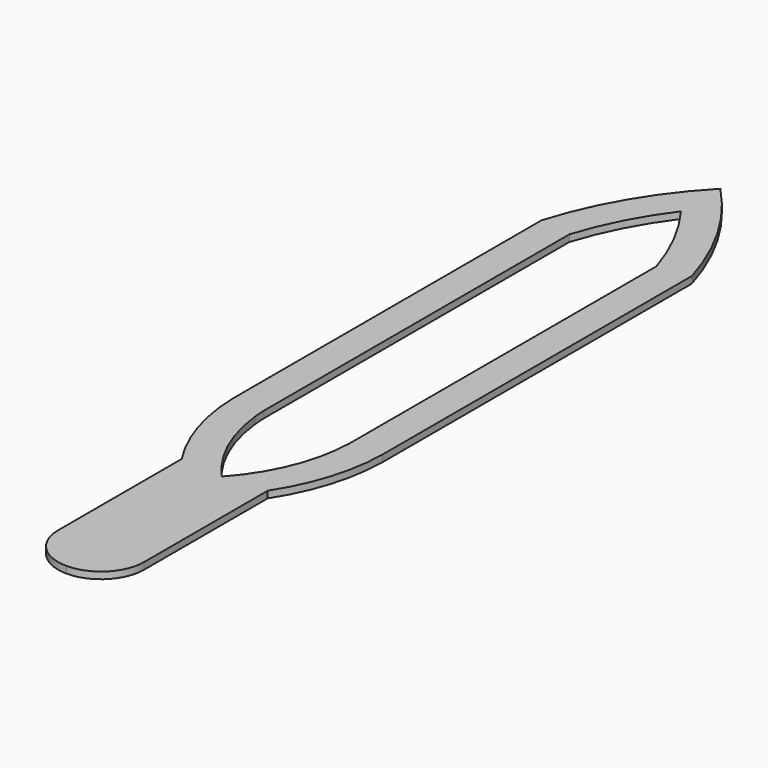
from build123d import *

# Parameters (mm, degrees)
F1_DEPTH = 4
F2_R     = 25.39999


# Not quite as in the source:
# - a fillet or chamfer is up to 0.001 mm smaller than in the source, because OpenCascade refuses the exact size


with BuildPart() as f1:
    # F0 (on Top) → F1 (new body)
    with BuildSketch(Plane.XY):
        with BuildLine():
            Line((25.4, 88.9), (25.4, 27.783106151))
            ThreePointArc((25.4, 27.783106151), (39.0875817391, 57.0211124393), (44.1814440725, 88.9))
            Line((44.1814440725, 88.9), (44.1814440725, 317.5))
            ThreePointArc((44.1814440725, 317.5), (26.6541395651, 358.2459104505), (0, 393.7))
            ThreePointArc((0, 393.7), (-26.9370466698, 358.2864987651), (-44.7185559275, 317.5))
            Line((-44.7185559275, 317.5), (-44.7185559275, 88.9))
            ThreePointArc((-44.7185559275, 88.9), (-39.2808523641, 57.0071475451), (-25.4, 27.783106151))
            Line((-25.4, 27.783106151), (-25.4, 81.8970223493))
            ThreePointArc((-25.4, 81.8970223493), (-25.7287156311, 85.5486031353), (-25.9225594861, 89.209821616))
            Line((-25.9225594861, 89.209821616), (-25.9225594861, 314.6655596019))
            ThreePointArc((-25.9225594861, 314.6655596019), (-15.1225925717, 340.7930484479), (-0.0869368678, 364.7349367673))
            ThreePointArc((-0.0869368678, 364.7349367673), (14.7574318658, 340.7960081036), (25.385447631, 314.7101331987))
            Line((25.385447631, 314.7101331987), (25.385447631, 89.0840377413))
            ThreePointArc((25.385447631, 89.0840377413), (25.3835184902, 88.992017936), (25.3815021522, 88.9))
            Line((25.3815021522, 88.9), (25.4, 88.9))
        make_face()
        with BuildLine():
            Line((-25.4, -88.9), (25.4, -88.9))
            Line((25.4, -88.9), (25.4, 27.783106151))
            ThreePointArc((25.4, 27.783106151), (13.8352633227, 12.8536673819), (0, 0))
            ThreePointArc((0, 0), (-13.8130547318, 12.8739710228), (-25.4, 27.783106151))
            Line((-25.4, 27.783106151), (-25.4, -88.9))
        make_face()
        with BuildLine():
            ThreePointArc((0, 0), (13.8352633227, 12.8536673819), (25.4, 27.783106151))
            Line((25.4, 27.783106151), (25.4, 88.9))
            Line((25.4, 88.9), (25.3815021522, 88.9))
            ThreePointArc((25.3815021522, 88.9), (18.4387554256, 54.950742752), (0.0203713554, 25.5991341412))
            ThreePointArc((0.0203713554, 25.5991341412), (-17.1734173627, 51.7235821598), (-25.4, 81.8970223493))
            Line((-25.4, 81.8970223493), (-25.4, 27.783106151))
            ThreePointArc((-25.4, 27.783106151), (-13.8130547318, 12.8739710228), (0, 0))
        make_face()
    extrude(amount=F1_DEPTH)

    # F2 (radius 25.4 in the source; OpenCascade refuses exactly that, so slightly less here)
    f2_edges = [f1.edges().sort_by_distance(p)[0] for p in [
        (-25.4, -88.9, 2),
        (25.4, -88.9, 2),
    ]]
    fillet(f2_edges, radius=F2_R)


solid = f1.part
